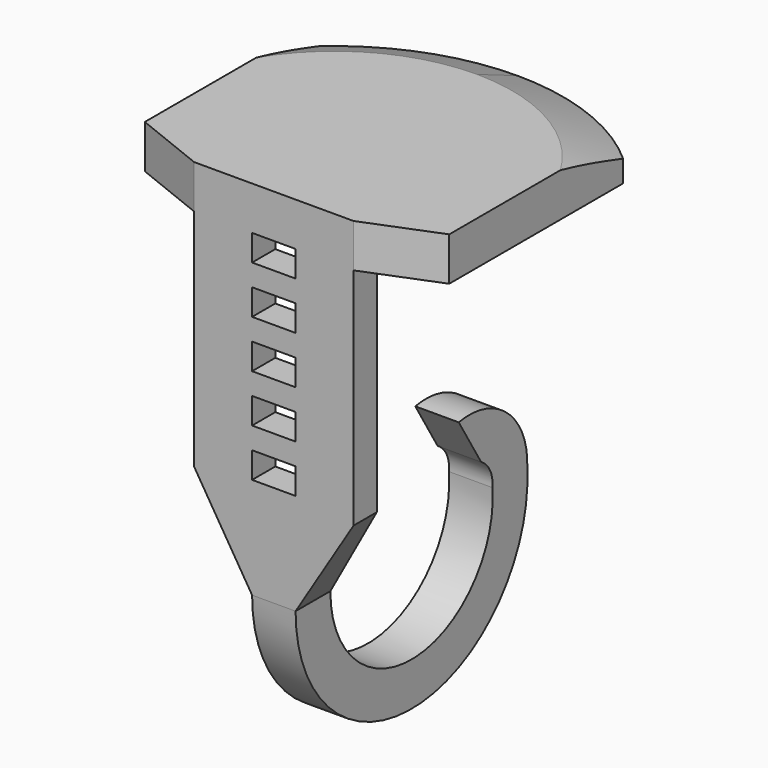
from build123d import *

# Parameters (mm, degrees)
F1_DEPTH    = 6
F2_W        = 8
F2_H        = 4
F3_DEPTH    = 36
F4_DEPTH    = 4
F5_C1_SIZE2 = 10
F5_C1_SIZE  = 4
F5_C2_SIZE2 = 10
F5_C2_SIZE  = 4
F6_W        = 4
F6_H        = 3
F7_DEPTH    = 6
F10_DEPTH   = 3
F11_W       = 14
F11_H       = 4
F11_W_2     = 8
F12_DEPTH   = 1
F12_FACE_W  = 22
F12_FACE_H  = 4
F10_FACE_W  = 6
F10_FACE_H  = 6
F15_DEPTH   = 109
F16_SIZE2   = 3
F16_SIZE    = 7


# Not quite as in the source:
# - an extrude ends at something that could not be found from the text; its depth is read off the source's solid


with BuildPart() as f1:
    # F0 (on Top) → F1 (new body)
    with BuildSketch(Plane.XY):
        with BuildLine():
            ThreePointArc((4.2292630374, 28.5867799968), (-5.5346345873, 34.5190491883), (-16.7707372875, 36.5867799968))
            ThreePointArc((-16.7707372875, 36.5867799968), (-28.0068396415, 34.5190490726), (-37.7707369626, 28.5867799968))
            Line((-37.7707369626, 28.5867799968), (-37.7707369626, -1.4132200032))
            Line((-37.7707369626, -1.4132200032), (4.2292630374, -1.4132200032))
            Line((4.2292630374, -1.4132200032), (4.2292630374, 28.5867799968))
        make_face()
    extrude(amount=F1_DEPTH)

    # F2 (on face) → F3 (join)
    with BuildSketch(Plane.XY.offset(6)):
        with Locations((-23.7707369626, -3.4132200032)):
            Rectangle(F2_W, F2_H)
        with Locations((-9.7707369626, -3.4132200032)):
            Rectangle(F2_W, F2_H)
    extrude(amount=-F3_DEPTH)

    # F4 (add): faces of the model
    f4_faces = [f1.faces().sort_by_distance(p)[0] for p in [
        (-32.7707369626, -1.4132200032, 3),
        (-0.7707369626, -1.4132200032, 3),
        (-16.7707369626, -1.4132200032, 3),
    ]]
    extrude(f4_faces, amount=F4_DEPTH)

    # F5: chamfer of 10 x 4 on 2 edges, made by hand

    # F5_c1
    f5_c1_edges = [f1.edges().sort_by_distance(p)[0] for p in [
        (-37.7707369626, -5.4132200032, 3),
    ]]
    f5_c1_side = f1.faces().sort_by_distance((-37.7707369626, -5.3332200032, 3))[0]
    chamfer(f5_c1_edges, length=F5_C1_SIZE, length2=F5_C1_SIZE2, reference=f5_c1_side)

    # F5_c2
    f5_c2_edges = [f1.edges().sort_by_distance(p)[0] for p in [
        (4.2292630374, -5.4132200032, 3),
    ]]
    f5_c2_side = f1.faces().sort_by_distance((4.2292630374, -5.3332200032, 3))[0]
    chamfer(f5_c2_edges, length=F5_C2_SIZE, length2=F5_C2_SIZE2, reference=f5_c2_side)

    # F6 (on face) → F7 (join, through all)
    with BuildSketch(Plane(origin=(-13.7707369626, 0, 0), x_dir=(0, -1, 0), z_dir=(-1, 0, 0))):
        with Locations((3.4132200032, -24.9)):
            Rectangle(F6_W, F6_H)
        with Locations((3.4132200032, -18.3)):
            Rectangle(F6_W, F6_H)
        with Locations((3.4132200032, -11.7)):
            Rectangle(F6_W, F6_H)
        with Locations((3.4132200032, -5.1)):
            Rectangle(F6_W, F6_H)
    extrude(amount=F7_DEPTH)

    # F11 (on face) → F12 (join)
    with BuildSketch(Plane(origin=(0, 0, -30), x_dir=(1, 0, 0), z_dir=(0, 0, -1))):
        with Locations((-12.7707369626, 3.4132200032)):
            Rectangle(F11_W, F11_H)
        with Locations((-23.7707369626, 3.4132200032)):
            Rectangle(F11_W_2, F11_H)
    extrude(amount=F12_DEPTH)



with BuildPart() as f10:
    # F9 (on line) → F10 (new body, symmetric)
    with BuildSketch(Plane.YZ.offset(-16.7707369626)):
        with BuildLine():
            ThreePointArc((-5.4132200032, -44), (15.1917157006, -63.9908492264), (34.5501852762, -42.7906821553))
            ThreePointArc((34.5501852762, -42.7906821553), (24.5246696764, -32.3338991708), (14.5746107682, -42.8625078704))
            Line((14.5746107682, -42.8625078704), (20.5957170737, -42.8625078704))
            ThreePointArc((20.5957170737, -42.8625078704), (24.5244376896, -38.3339982315), (28.5344518581, -42.7906821553))
            ThreePointArc((28.5344518581, -42.7906821553), (15.1920047243, -57.9869118475), (0.5867799968, -44))
            Line((0.5867799968, -44), (-5.4132200032, -44))
        make_face()
    extrude(amount=F10_DEPTH, both=True)


with BuildPart() as f1_1:
    add(f1.part)

    add(f10.part)  # F13 merges F10
    # F12_face (on face) → F13 section 0
    with BuildSketch(Plane(origin=(-16.7707369626, -3.4132200032, -31), x_dir=(1, 0, 0), z_dir=(0, 0, -1))):
        Rectangle(F12_FACE_W, F12_FACE_H)
    # F10_face (on face) → F13 section 1
    with BuildSketch(Plane(origin=(-16.7707369626, -2.4132200032, -44), x_dir=(1, 0, 0), z_dir=(0, 0, 1))):
        Rectangle(F10_FACE_W, F10_FACE_H)
    loft()

    # F14 (on face) → F15 (cut, through all)
    with BuildSketch(Plane.YZ.offset(-13.7707369626)):
        with BuildLine():
            Line((22.7304068946, -32.502746223), (21.8552816659, -31.0546644032))
            Line((21.8552816659, -31.0546644032), (14.088241172, -33.6755602773))
            Line((14.088241172, -33.6755602773), (14.5746107682, -42.8625078704))
            ThreePointArc((14.5746107682, -42.8625078704), (16.7033355644, -36.1481265127), (22.7304068946, -32.502746223))
        make_face()
        with BuildLine():
            Line((26.5877404927, -38.885529479), (22.7304068946, -32.502746223))
            ThreePointArc((22.7304068946, -32.502746223), (16.7033355644, -36.1481265127), (14.5746107682, -42.8625078704))
            Line((14.5746107682, -42.8625078704), (20.5957170737, -42.8625078704))
            ThreePointArc((20.5957170737, -42.8625078704), (22.3486471202, -39.0010956404), (26.5877404927, -38.885529479))
        make_face()
    extrude(amount=-F15_DEPTH, mode=Mode.SUBTRACT)

    # F16
    f16_edges = [f1_1.edges().sort_by_distance(p)[0] for p in [
        (-16.770737, 36.58678, 6),
    ]]
    f16_side = f1_1.faces().sort_by_distance((-16.770737, 14.854781, 6))[0]
    chamfer(f16_edges, length=F16_SIZE, length2=F16_SIZE2, reference=f16_side)


solid = f1_1.part
